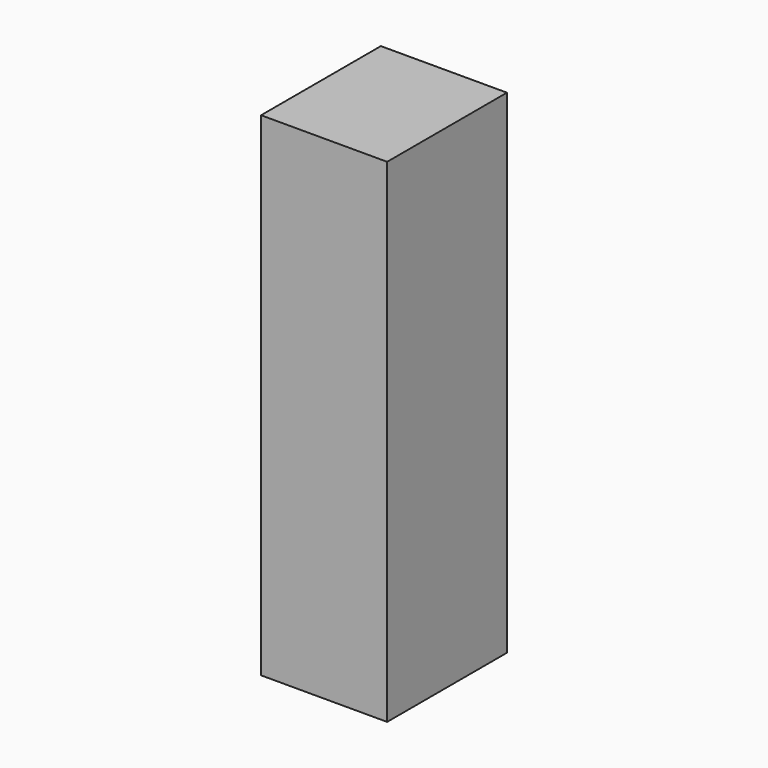
from build123d import *

# Parameters (mm, degrees)
F0_W     = 42.7710562944
F0_H     = 167.2781854868
F1_DEPTH = 50.8


# Not quite as in the source:
# - a feature of the source that left no trace in its solid (it failed there, or was rolled back) is left out


with BuildPart() as f1:
    # F0 (on Front) → F1 (new body)
    with BuildSketch(Plane.XZ):
        Rectangle(F0_W, F0_H)
    extrude(amount=-F1_DEPTH)


solid = f1.part
